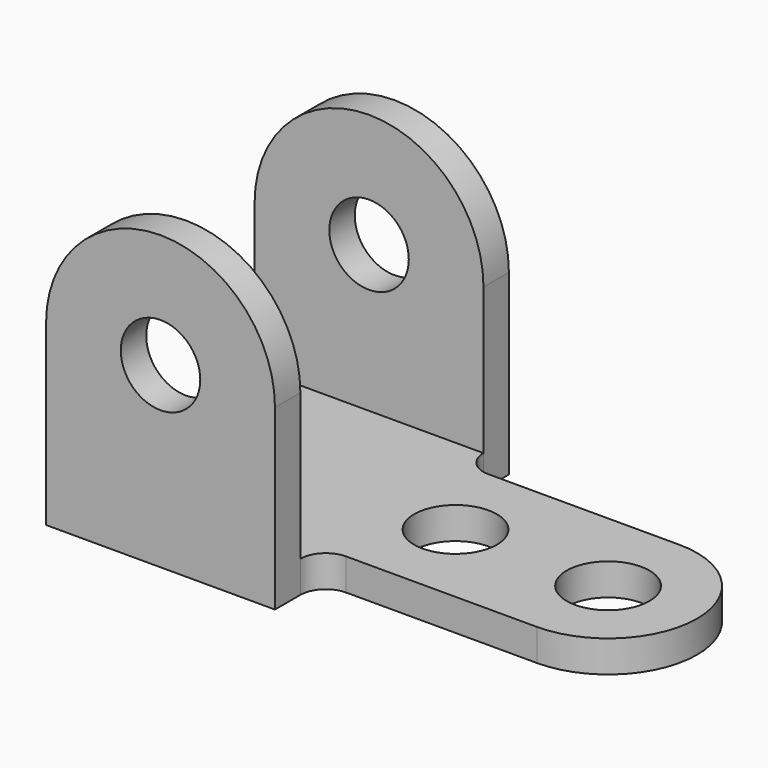
from build123d import *

# Parameters (mm, degrees)
F0_R     = 10.3251
F1_DEPTH = 7.9375
F2_R     = 9.92251
F3_DEPTH = 7.9375
F4_R     = 6.35


# Not quite as in the source:
# - a pattern or mirror of a feature is missing from the dataset's text; its kind, count and spacing are read off the source's solid


with BuildPart() as f1:
    # F0 (on Top) → F1 (new body)
    with BuildSketch(Plane.XY):
        with BuildLine():
            Line((0, 73.025), (0, 0))
            Line((0, 0), (57.15, 0))
            Line((57.15, 0), (57.15, 14.2875))
            Line((57.15, 14.2875), (111.125, 14.2875))
            ThreePointArc((111.125, 14.2875), (133.35, 36.5125), (111.125, 58.7375))
            Line((111.125, 58.7375), (57.15, 58.7375))
            Line((57.15, 58.7375), (57.15, 73.025))
            Line((57.15, 73.025), (0, 73.025))
        make_face()
        with Locations((73.025, 36.5125)):
            Circle(F0_R, mode=Mode.SUBTRACT)
        with Locations((111.125, 36.5125)):
            Circle(F0_R, mode=Mode.SUBTRACT)
    extrude(amount=F1_DEPTH)

    # F2 (on Front) → F3 (join)
    with BuildSketch(Plane.XZ):
        with BuildLine():
            Line((0, 44.45), (0, 0))
            Line((0, 0), (57.15, 0))
            Line((57.15, 0), (57.15, 44.45))
            ThreePointArc((57.15, 44.45), (28.575, 73.025), (0, 44.45))
        make_face()
        with Locations((28.575, 44.45)):
            Circle(F2_R, mode=Mode.SUBTRACT)
    f3 = extrude(amount=-F3_DEPTH)

    # F3_copies: F3 across plane
    add(f3.mirror(Plane.ZX.offset(36.5125)))

    # F4
    f4_edges = [f1.edges().sort_by_distance(p)[0] for p in [
        (57.15, 14.2875, 3.96875),
        (57.15, 58.7375, 3.96875),
    ]]
    fillet(f4_edges, radius=F4_R)


solid = f1.part
